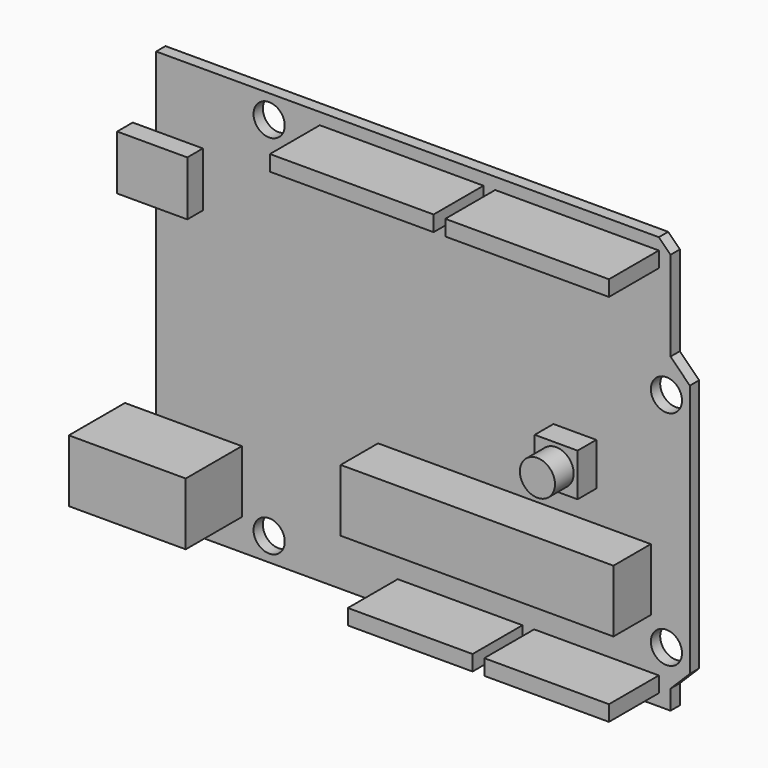
from build123d import *

# Parameters (mm, degrees)
F0_R          = 2
F1_DEPTH      = 1.5
F2_W          = 21
F2_H          = 2
F2_W_2        = 16
F2_H_2        = 1.9774034154
F3_DEPTH      = 8
F4_W          = 11
F4_H          = 8
F5_DEPTH      = 9
F7_DEPTH      = 4
F8_W          = 6
F8_H          = 7
F9_DEPTH      = 2.5
F10_W         = 2.5
F10_H         = 7
F11_DEPTH     = 3
F12_TEXT_SIZE = 6.9444444444
F13_DEPTH     = 0.1
F14_W         = 35
F14_H         = 8
F15_DEPTH     = 6
F16_W         = 5.5
F16_H         = 5.5
F17_DEPTH     = 3
F18_R         = 2.25
F19_DEPTH     = 3


# Not quite as in the source:
# - Text() gives the source's letters only with a copy of the font that has no kerning and outlines rounded to 1/6400 em; it was checked with that copy


with BuildPart() as f1:
    # F0 (on Front) → F1 (new body)
    with BuildSketch(Plane.XZ):
        Polygon((0, 53), (0, 0), (66, 0), (66, 2.5), (68.4748737342, 4.9748737342), (68.4748737342, 37.5251262658), (66, 40), (66, 49.5), (66, 51.5), (64.5, 53), align=None)
        with Locations((14.5, 3)):
            Circle(F0_R, mode=Mode.SUBTRACT)
        with Locations((65.4748737342, 6.9802752385)):
            Circle(F0_R, mode=Mode.SUBTRACT)
        with Locations((14.5, 50)):
            Circle(F0_R, mode=Mode.SUBTRACT)
        with Locations((65.4748737342, 35.5086197467)):
            Circle(F0_R, mode=Mode.SUBTRACT)
    extrude(amount=F1_DEPTH)

    # F2 (on face) → F3 (join)
    with BuildSketch(Plane.XZ.offset(1.5)):
        with Locations((54, 50.5)):
            Rectangle(F2_W, F2_H)
        with Locations((31.5, 50.5)):
            Rectangle(F2_W, F2_H)
        with Locations((56.5, 2.5)):
            Rectangle(F2_W_2, F2_H)
        with Locations((39, 2.4887017077)):
            Rectangle(F2_W_2, F2_H_2)
    extrude(amount=F3_DEPTH)

    # F4 (on face) → F5 (join)
    with BuildSketch(Plane.XZ.offset(1.5)):
        with Locations((5.5, 8)):
            Rectangle(F4_W, F4_H)
    extrude(amount=F5_DEPTH)

    # F6 (on face) → F7 (join)
    with BuildSketch(Plane(origin=(0, 0, 0), x_dir=(0, -1, 0), z_dir=(-1, 0, 0))):
        with BuildLine():
            Line((10.5, 4), (10.5, 12))
            Line((10.5, 12), (6.5, 12))
            Line((6.5, 12), (6.5, 10.75))
            ThreePointArc((6.5, 10.75), (8.4445436483, 9.9445436483), (9.25, 8))
            ThreePointArc((9.25, 8), (8.4445436483, 6.0554563517), (6.5, 5.25))
            Line((6.5, 5.25), (6.5, 4))
            Line((6.5, 4), (10.5, 4))
        make_face()
        with BuildLine():
            Line((6.5, 10.75), (6.5, 12))
            Line((6.5, 12), (1.5, 12))
            Line((1.5, 12), (1.5, 4))
            Line((1.5, 4), (6.5, 4))
            Line((6.5, 4), (6.5, 5.25))
            ThreePointArc((6.5, 5.25), (3.75, 8), (6.5, 10.75))
        make_face()
    extrude(amount=F7_DEPTH)

    # F8 (on face) → F9 (join)
    with BuildSketch(Plane.XZ.offset(1.5)):
        with Locations((3, 40.5)):
            Rectangle(F8_W, F8_H)
    extrude(amount=F9_DEPTH)

    # F10 (on face) → F11 (join)
    with BuildSketch(Plane(origin=(0, 0, 0), x_dir=(0, -1, 0), z_dir=(-1, 0, 0))):
        with Locations((2.75, 40.5)):
            Rectangle(F10_W, F10_H)
        Polygon((2.5, 43.5), (3.5, 43.5), (3.5, 37.5), (2.5, 37.5), (2, 38), (2, 43), align=None, mode=Mode.SUBTRACT)
    extrude(amount=F11_DEPTH)

    # F12 (on face) → F13 (join)
    with BuildSketch(Plane(origin=(0, 0, 0), x_dir=(-1, 0, 0), z_dir=(0, 1, 0))):
        with Locations((-60, 43)):
            Text('Adam Ardeishar', F12_TEXT_SIZE, font='Open Sans', text_align=(TextAlign.LEFT, TextAlign.BOTTOM))
        with Locations((-60, 33)):
            Text('Andrew Nam', F12_TEXT_SIZE, font='Open Sans', text_align=(TextAlign.LEFT, TextAlign.BOTTOM))
    extrude(amount=F13_DEPTH)

    # F14 (on face) → F15 (join)
    with BuildSketch(Plane.XZ.offset(1.5)):
        with Locations((45.9748737342, 14)):
            Rectangle(F14_W, F14_H)
    extrude(amount=F15_DEPTH)

    # F16 (on face) → F17 (join)
    with BuildSketch(Plane.XZ.offset(1.5)):
        with Locations((53.7248737342, 24.75)):
            Rectangle(F16_W, F16_H)
    extrude(amount=F17_DEPTH)

    # F18 (on face) → F19 (join)
    with BuildSketch(Plane.XZ.offset(4.5)):
        with Locations((53.7248737342, 24.75)):
            Circle(F18_R)
    extrude(amount=F19_DEPTH)


solid = f1.part
